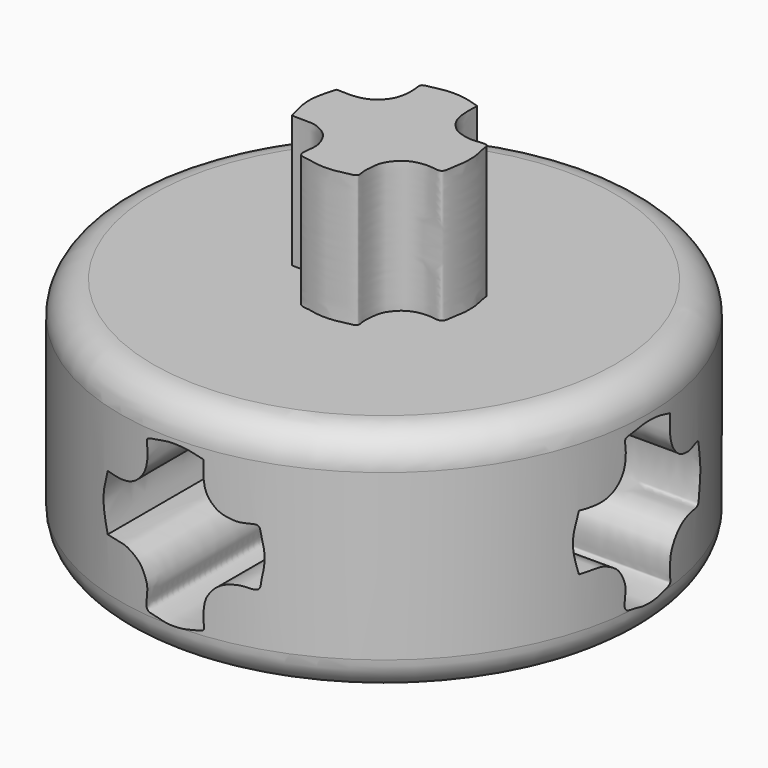
from build123d import *

# Parameters (mm, degrees)
F0_R          = 8
F1_DEPTH      = 7
F3_DEPTH      = 4
F5_DEPTH      = 25
F5_DEPTH_BACK = 25
F7_DEPTH      = 25
F7_DEPTH_BACK = 25


# Not quite as in the source:
# - a fillet or chamfer that OpenCascade refuses, or shapes differently, is made with other operations: its cross-section is extruded or revolved along the edge and cut away or added


with BuildPart() as f1:
    # F0 (on Top) → F1 (new body)
    with BuildSketch(Plane.XY):
        Circle(F0_R)
    extrude(amount=F1_DEPTH)

    # F2 (on face) → F3 (join)
    with BuildSketch(Plane.XY.offset(7)):
        with BuildLine():
            add(Edge.make_bspline(
                [(-2.1453189292, -0.812403534), (-2.2291799027, -0.5147854162), (-2.3965988205, 0.0693154166), (-2.2270661408, 0.6183251281), (-2.1453189292, 0.8875972993)],
                knots=[0, 0, 0, 0, 0.5095712537, 1, 1, 1, 1], degree=3))
            add(Edge.make_bspline(
                [(-2.1453189292, -0.812403534), (-2.0462146869, -0.812546633), (-1.8562976232, -0.8128208589), (-1.5995258635, -0.8109702484), (-1.4107650431, -0.8271952097), (-1.0525308973, -0.9991228135), (-0.881515203, -1.2019496068), (-0.7462403154, -1.4790785152), (-0.6941521408, -1.7721486922), (-0.8264550317, -2.3060372512), (-0.4252380891, -2.3094553952), (-0.1641394597, -2.39328354), (0.171847139, -2.4065584213), (0.4619958492, -2.3819187352), (0.7053356837, -2.3086277115), (1.0355815173, -2.2738283861), (0.9578656682, -2.0264843097), (0.972329852, -1.7262282264), (1.0043166569, -1.4743095735), (1.0802938039, -1.2844806936), (1.2606264856, -1.0560642251), (1.4022161443, -0.9536037149), (1.5820445887, -0.8553488053), (1.8405387734, -0.8091796541), (2.0652910938, -0.7963302445), (2.4574534093, -0.8884051228), (2.4647792182, -0.5364288415), (2.5502262108, -0.2130675085), (2.5516869242, 0.0734966508), (2.5466202723, 0.3368604343), (2.4464405951, 0.6869113476), (2.4458836528, 0.9477445076), (2.0587086229, 0.8750622393), (1.8110087922, 0.8774528734), (1.460553932, 0.9794284484), (1.2720689076, 1.1213458505), (1.039296652, 1.3914645052), (0.9576696828, 1.8177575628), (0.969636174, 2.1409695187), (0.9758471819, 2.3087272993)],
                knots=[0, 0, 0, 0, 0.0273605905, 0.0524320947, 0.0745076412, 0.1056108167, 0.1318649214, 0.158948127, 0.1874687016, 0.220995097, 0.2482860623, 0.2755720453, 0.3045111481, 0.3315301836, 0.3578655515, 0.3837385363, 0.4059679792, 0.434252013, 0.4594532962, 0.4822711791, 0.5090972104, 0.530231005, 0.5527300135, 0.5781274322, 0.6031996615, 0.6315546276, 0.6576667534, 0.6876672756, 0.714256594, 0.7402463844, 0.7710533559, 0.7932728015, 0.8216277676, 0.8482190477, 0.8777914221, 0.9023565188, 0.9315770045, 0.9644861842, 1, 1, 1, 1], degree=3))
            add(Edge.make_bspline(
                [(-2.1453189292, 0.8875972993), (-1.9521964497, 0.8780475085), (-1.5848074134, 0.8603693676), (-1.1304602567, 0.9960226139), (-0.8202192306, 1.3400161654), (-0.7149185223, 1.6828007485), (-0.70557119, 2.0923268409), (-0.7793227574, 2.3463238004), (-0.4576002352, 2.3842425435), (-0.1008664347, 2.4800264396), (0.2451665152, 2.4783343449), (0.5684540927, 2.4417658867), (0.8334725478, 2.3546593956), (0.9758471819, 2.3087272993)],
                knots=[0, 0, 0, 0, 0.1117445823, 0.2125923647, 0.3107430927, 0.4000660841, 0.4960442665, 0.5626441507, 0.6379036869, 0.7311412958, 0.8178947498, 0.9022950941, 1, 1, 1, 1], degree=3))
        make_face()
    extrude(amount=F3_DEPTH)

    # F4 (on Right) → F5 (cut, two sides)
    with BuildSketch(Plane.YZ) as f5_sk:
        with BuildLine():
            add(Edge.make_bspline(
                [(-2.2211652576, 2.5211653882), (-2.3050262311, 2.8187835061), (-2.4724451489, 3.4028843389), (-2.3029124692, 3.9518940503), (-2.2211652576, 4.2211662216)],
                knots=[0, 0, 0, 0, 0.5095712537, 1, 1, 1, 1], degree=3))
            add(Edge.make_bspline(
                [(-2.2211652576, 2.5211653882), (-2.1220610153, 2.5210222892), (-1.9321439516, 2.5207480634), (-1.6753721919, 2.5225986738), (-1.4866113715, 2.5063737125), (-1.1283772257, 2.3344461087), (-0.9573615314, 2.1316193155), (-0.8220866438, 1.854490407), (-0.7699984692, 1.56142023), (-0.9023013601, 1.0275316711), (-0.5010844175, 1.024113527), (-0.2399857881, 0.9402853822), (0.0960008106, 0.927010501), (0.3861495208, 0.951650187), (0.6294893553, 1.0249412107), (0.9597351889, 1.0597405361), (0.8820193398, 1.3070846125), (0.8964835236, 1.6073406958), (0.9284703285, 1.8592593487), (1.0044474755, 2.0490882286), (1.1847801572, 2.2775046971), (1.3263698159, 2.3799652073), (1.5061982603, 2.478220117), (1.764692445, 2.5243892682), (1.9894447654, 2.5372386778), (2.3816070809, 2.4451637994), (2.3889328898, 2.7971400808), (2.4743798824, 3.1205014137), (2.4758405958, 3.4070655731), (2.4707739439, 3.6704293566), (2.3705942667, 4.0204802698), (2.3700373244, 4.2813134299), (1.9828622945, 4.2086311615), (1.7351624638, 4.2110217957), (1.3847076036, 4.3129973707), (1.1962225792, 4.4549147728), (0.9634503236, 4.7250334274), (0.8818233544, 5.1513264851), (0.8937898456, 5.4745384409), (0.9000008535, 5.6422962216)],
                knots=[0, 0, 0, 0, 0.0273605905, 0.0524320947, 0.0745076412, 0.1056108167, 0.1318649214, 0.158948127, 0.1874687016, 0.220995097, 0.2482860623, 0.2755720453, 0.3045111481, 0.3315301836, 0.3578655515, 0.3837385363, 0.4059679792, 0.434252013, 0.4594532962, 0.4822711791, 0.5090972104, 0.530231005, 0.5527300135, 0.5781274322, 0.6031996615, 0.6315546276, 0.6576667534, 0.6876672756, 0.714256594, 0.7402463844, 0.7710533559, 0.7932728015, 0.8216277676, 0.8482190477, 0.8777914221, 0.9023565188, 0.9315770045, 0.9644861842, 1, 1, 1, 1], degree=3))
            add(Edge.make_bspline(
                [(-2.2211652576, 4.2211662216), (-2.0280427781, 4.2116164307), (-1.6606537418, 4.1939382898), (-1.2063065851, 4.3295915362), (-0.896065559, 4.6735850876), (-0.7907648507, 5.0163696708), (-0.7814175184, 5.4258957632), (-0.8551690858, 5.6798927226), (-0.5334465636, 5.7178114657), (-0.1767127631, 5.8135953618), (0.1693201868, 5.8119032671), (0.4926077643, 5.775334809), (0.7576262194, 5.6882283179), (0.9000008535, 5.6422962216)],
                knots=[0, 0, 0, 0, 0.1117445823, 0.2125923647, 0.3107430927, 0.4000660841, 0.4960442665, 0.5626441507, 0.6379036869, 0.7311412958, 0.8178947498, 0.9022950941, 1, 1, 1, 1], degree=3))
        make_face()
    extrude(amount=-F5_DEPTH, mode=Mode.SUBTRACT)
    extrude(f5_sk.sketch, amount=F5_DEPTH_BACK, mode=Mode.SUBTRACT)

    # F6 (on Front) → F7 (cut, two sides)
    with BuildSketch(Plane.XZ) as f7_sk:
        with BuildLine():
            add(Edge.make_bspline(
                [(-2.2311653919, 2.5852779835), (-2.3150263655, 2.8828961014), (-2.4824452833, 3.4669969342), (-2.3129126036, 4.0160066456), (-2.2311653919, 4.2852788168)],
                knots=[0, 0, 0, 0, 0.5095712537, 1, 1, 1, 1], degree=3))
            add(Edge.make_bspline(
                [(-2.2311653919, 2.5852779835), (-2.1320611497, 2.5851348845), (-1.942144086, 2.5848606586), (-1.6853723262, 2.5867112691), (-1.4966115058, 2.5704863078), (-1.13837736, 2.398558704), (-0.9673616658, 2.1957319107), (-0.8320867781, 1.9186030023), (-0.7799986035, 1.6255328253), (-0.9123014945, 1.0916442664), (-0.5110845519, 1.0882261223), (-0.2499859225, 1.0043979775), (0.0860006762, 0.9911230963), (0.3761493864, 1.0157627823), (0.619489221, 1.089053806), (0.9497350545, 1.1238531314), (0.8720192055, 1.3711972078), (0.8864833893, 1.6714532911), (0.9184701942, 1.923371944), (0.9944473412, 2.1132008239), (1.1747800229, 2.3416172924), (1.3163696815, 2.4440778026), (1.496198126, 2.5423327122), (1.7546923106, 2.5885018635), (1.979444631, 2.6013512731), (2.3716069465, 2.5092763947), (2.3789327554, 2.8612526761), (2.464379748, 3.184614009), (2.4658404614, 3.4711781683), (2.4607738096, 3.7345419519), (2.3605941323, 4.0845928651), (2.3600371901, 4.3454260251), (1.9728621602, 4.2727437568), (1.7251623295, 4.275134391), (1.3747074692, 4.377109966), (1.1862224448, 4.5190273681), (0.9534501893, 4.7891460227), (0.8718232201, 5.2154390804), (0.8837897113, 5.5386510362), (0.8900007192, 5.7064088168)],
                knots=[0, 0, 0, 0, 0.0273605905, 0.0524320947, 0.0745076412, 0.1056108167, 0.1318649214, 0.158948127, 0.1874687016, 0.220995097, 0.2482860623, 0.2755720453, 0.3045111481, 0.3315301836, 0.3578655515, 0.3837385363, 0.4059679792, 0.434252013, 0.4594532962, 0.4822711791, 0.5090972104, 0.530231005, 0.5527300135, 0.5781274322, 0.6031996615, 0.6315546276, 0.6576667534, 0.6876672756, 0.714256594, 0.7402463844, 0.7710533559, 0.7932728015, 0.8216277676, 0.8482190477, 0.8777914221, 0.9023565188, 0.9315770045, 0.9644861842, 1, 1, 1, 1], degree=3))
            add(Edge.make_bspline(
                [(-2.2311653919, 4.2852788168), (-2.0380429125, 4.275729026), (-1.6706538762, 4.2580508851), (-1.2163067194, 4.3937041315), (-0.9060656934, 4.7376976829), (-0.8007649851, 5.080482266), (-0.7914176528, 5.4900083584), (-0.8651692201, 5.7440053179), (-0.5434466979, 5.781924061), (-0.1867128974, 5.8777079571), (0.1593200525, 5.8760158624), (0.4826076299, 5.8394474043), (0.7476260851, 5.7523409132), (0.8900007192, 5.7064088168)],
                knots=[0, 0, 0, 0, 0.1117445823, 0.2125923647, 0.3107430927, 0.4000660841, 0.4960442665, 0.5626441507, 0.6379036869, 0.7311412958, 0.8178947498, 0.9022950941, 1, 1, 1, 1], degree=3))
        make_face()
    extrude(amount=-F7_DEPTH, mode=Mode.SUBTRACT)
    extrude(f7_sk.sketch, amount=F7_DEPTH_BACK, mode=Mode.SUBTRACT)

    # F8: fillet of radius 1 on 2 edges, made by hand

    # F8_s1 → F8_t2 (revolve, cut)
    with BuildSketch(Plane.XZ):
        with BuildLine():
            ThreePointArc((8, 1), (7.7071067812, 0.2928932188), (7, 0))
            Line((7, 0), (8, 0))
            Line((8, 0), (8, 1))
        make_face()
    revolve(axis=Axis((0, 0, 0), (0, 0, 1)), mode=Mode.SUBTRACT)

    # F8_s3 → F8_t4 (revolve, cut)
    with BuildSketch(Plane.XZ):
        with BuildLine():
            ThreePointArc((8, 6), (7.7071067812, 6.7071067812), (7, 7))
            Line((7, 7), (8, 7))
            Line((8, 7), (8, 6))
        make_face()
    revolve(axis=Axis((0, 0, 7), (0, 0, 1)), mode=Mode.SUBTRACT)


solid = f1.part
